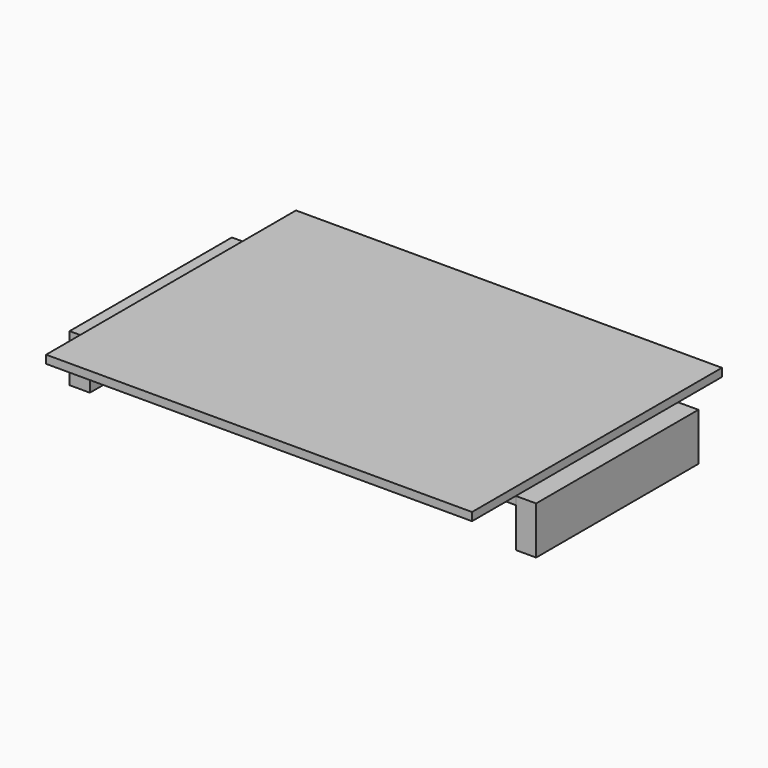
from build123d import *

# Parameters (mm, degrees)
F0_W     = 105
F0_H     = 77
F0_W_2   = 5
F0_H_2   = 50
F2_DEPTH = 2
F1_W     = 5
F1_H     = 50
F3_DEPTH = 11.75
F1_W_2   = 20
F1_W_3   = 8.9916351438
F1_W_4   = 6.0083648562
F4_DEPTH = 2


with BuildPart() as f2:
    # F0 (on Top) → F2 (new body)
    with BuildSketch(Plane.XY):
        Rectangle(F0_W, F0_H)
        with Locations((43.9916351438, 0)):
            Rectangle(F0_W_2, F0_H_2, mode=Mode.SUBTRACT)
        with Locations((43.9916351438, 0)):
            Rectangle(F0_W_2, F0_H_2)
    extrude(amount=F2_DEPTH)

    # F1 (on face) + F0 (on Top) → F4 (join)
    with BuildSketch(Plane.XY):
        with Locations((-42.5, 0)):
            Rectangle(F1_W_2, F1_H)
        with Locations((36.9958175719, 0)):
            Rectangle(F1_W_3, F1_H)
        with Locations((49.4958175719, 0)):
            Rectangle(F1_W_4, F1_H)
    with BuildSketch(Plane.XY):
        with Locations((43.9916351438, 0)):
            Rectangle(F0_W_2, F0_H_2)
    extrude(amount=-F4_DEPTH)


with BuildPart() as f3:
    # F1 (on face) → F3 (new body)
    with BuildSketch(Plane.XY):
        with Locations((-55, 0)):
            Rectangle(F1_W, F1_H)
    extrude(amount=-F3_DEPTH)


with BuildPart() as f3b:
    # F1 (on face) → F3, piece 2 (new body)
    with BuildSketch(Plane.XY):
        with Locations((55, 0)):
            Rectangle(F1_W, F1_H)
    extrude(amount=-F3_DEPTH)


solid = Compound([f2.part, f3.part, f3b.part])
